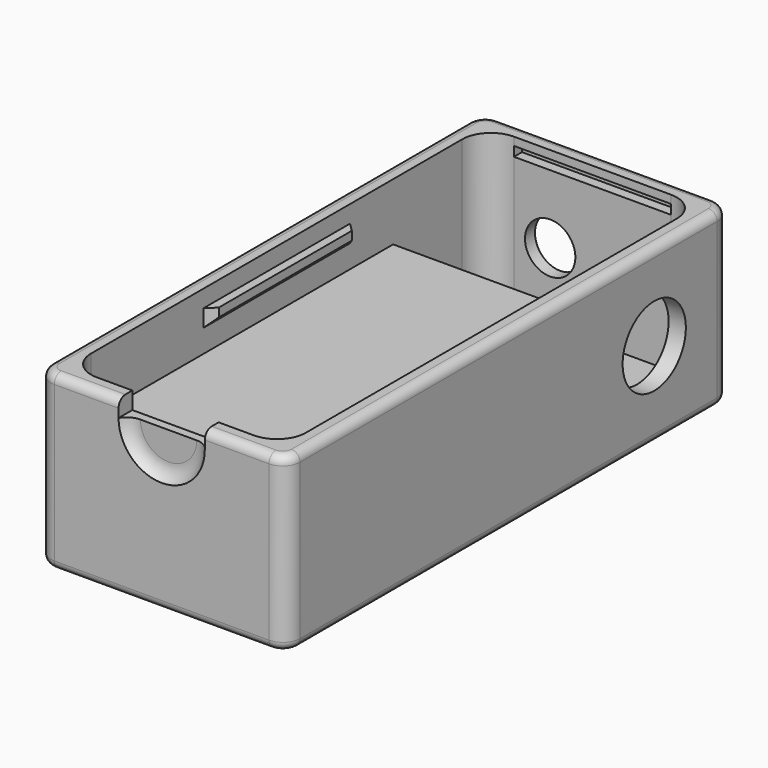
from build123d import *

# Parameters (mm, degrees)
F2_W         = 52
F2_H         = 116
F2_W_2       = 44.8
F2_H_2       = 108.8
F3_DEPTH     = 36
F4_DEPTH     = 3.6
F7_R         = 3.6
F8_R         = 5.9976
F6_R         = 5.25
F9_DEPTH     = 3.6
F5_R         = 8.25
F10_DEPTH    = 3.6
F11_W        = 18
F11_H        = 3.6
F12_DEPTH    = 3.6
F13_W        = 32.8048
F13_H        = 2
F14_DEPTH    = 2.1
F15_R        = 1.8
F6_R_2       = 12
F17_DEPTH    = 1
F18_R        = 0.5
F19_W        = 38.28
F19_H        = 3.6
F21_DEPTH    = 1.8
F20_W        = 38.28
F20_H        = 3.6
F22_DEPTH    = 1.8
F23_SIZE     = 1.79999
F25_DEPTH    = 1.8
F26_T2_ANGLE = 180
F27_W        = 41
F27_H        = 78
F28_DEPTH    = 22


# Not quite as in the source:
# - a fillet or chamfer that OpenCascade refuses, or shapes differently, is made with other operations: its cross-section is extruded or revolved along the edge and cut away or added
# - a fillet or chamfer is up to 0.001 mm smaller than in the source, because OpenCascade refuses the exact size
# - a feature of the source that left no trace in its solid (it failed there, or was rolled back) is left out


with BuildPart() as f3:
    # F2 (on Top) → F3 (new body)
    with BuildSketch(Plane.XY):
        Rectangle(F2_W, F2_H)
        Rectangle(F2_W_2, F2_H_2, mode=Mode.SUBTRACT)
    extrude(amount=F3_DEPTH)

    # F2 (on Top) → F4 (join)
    with BuildSketch(Plane.XY):
        Rectangle(F2_W_2, F2_H_2)
    extrude(amount=F4_DEPTH)

    # F7
    f7_edges = [f3.edges().sort_by_distance(p)[0] for p in [
        (26, 58, 18),
        (-26, 58, 18),
        (-26, -58, 18),
        (26, -58, 18),
    ]]
    fillet(f7_edges, radius=F7_R)

    # F8
    f8_edges = [f3.edges().sort_by_distance(p)[0] for p in [
        (-22.4, -54.4, 19.8),
        (22.4, -54.4, 19.8),
        (22.4, 54.4, 19.8),
        (-22.4, 54.4, 19.8),
    ]]
    fillet(f8_edges, radius=F8_R)

    # F6 (on face) → F9 (cut)
    with BuildSketch(Plane(origin=(0, 58, 0), x_dir=(-1, 0, 0), z_dir=(0, 1, 0))):
        with Locations((8.84, 18)):
            Circle(F6_R)
    extrude(amount=-F9_DEPTH, mode=Mode.SUBTRACT)

    # F5 (on face) → F10 (cut)
    with BuildSketch(Plane.YZ.offset(26)):
        with Locations((38, 18)):
            Circle(F5_R)
    extrude(amount=-F10_DEPTH, mode=Mode.SUBTRACT)

    # F11 (on face) → F12 (cut)
    with BuildSketch(Plane.XZ.offset(58)):
        with Locations((0, 34.2)):
            Rectangle(F11_W, F11_H)
    extrude(amount=-F12_DEPTH, mode=Mode.SUBTRACT)

    # F13 (on face) → F14 (cut)
    with BuildSketch(Plane.XZ.offset(-54.4)):
        with Locations((0, 33.3)):
            Rectangle(F13_W, F13_H)
    extrude(amount=-F14_DEPTH, mode=Mode.SUBTRACT)

    # F15
    f15_edges = [f3.edges().sort_by_distance(p)[0] for p in [
        (15.7, -58, 36),
        (24.945584, -56.945584, 36),
        (26, 0, 36),
        (-15.7, -58, 36),
        (-24.945584, -56.945584, 36),
        (-26, 0, 36),
        (-24.945584, 56.945584, 36),
        (0, 58, 36),
        (24.945584, 56.945584, 36),
        (0, -58, 0),
        (-24.945584, -56.945584, 0),
        (-26, 0, 0),
        (-24.945584, 56.945584, 0),
        (0, 58, 0),
        (24.945584, 56.945584, 0),
        (26, 0, 0),
        (24.945584, -56.945584, 0),
    ]]
    fillet(f15_edges, radius=F15_R)

    # F6 (on face) → F17 (cut)
    with BuildSketch(Plane(origin=(0, 58, 0), x_dir=(-1, 0, 0), z_dir=(0, 1, 0))):
        with Locations((8.84, 18)):
            Circle(F6_R_2)
        with Locations((8.84, 18)):
            Circle(F6_R, mode=Mode.SUBTRACT)
    extrude(amount=-F17_DEPTH, mode=Mode.SUBTRACT)

    # F18
    f18_edges = [f3.edges().sort_by_distance(p)[0] for p in [
        (0, 56.5, 34.3),
    ]]
    fillet(f18_edges, radius=F18_R)

    # F19 (on face) → F21 (join)
    with BuildSketch(Plane(origin=(22.4, 0, 0), x_dir=(0, -1, 0), z_dir=(-1, 0, 0))):
        with Locations((0, 30.6)):
            Rectangle(F19_W, F19_H)
    extrude(amount=F21_DEPTH)

    # F20 (on face) → F22 (join)
    with BuildSketch(Plane.YZ.offset(-22.4)):
        with Locations((0, 30.6)):
            Rectangle(F20_W, F20_H)
    extrude(amount=F22_DEPTH)

    # F23 (size 1.8 in the source; OpenCascade refuses exactly that, so slightly less here)
    f23_edges = [f3.edges().sort_by_distance(p)[0] for p in [
        (-20.6, -19.14, 30.6),
        (-20.6, 0, 28.8),
        (-20.6, 19.14, 30.6),
        (20.6, 19.14, 30.6),
        (20.6, 0, 28.8),
        (20.6, -19.14, 30.6),
    ]]
    chamfer(f23_edges, length=F23_SIZE)

    # F11 (on face) → F25 (cut)
    with BuildSketch(Plane.XZ.offset(58)):
        with BuildLine():
            ThreePointArc((-9, 32.4), (0, 23.4), (9, 32.4))
            Line((9, 32.4), (-9, 32.4))
        make_face()
    extrude(amount=-F25_DEPTH, mode=Mode.SUBTRACT)

    # F26: fillet of radius 3.6 on 1 edges, made by hand

    # F26_s1 → F26_t2 (revolve)
    with BuildSketch(Plane.XY.offset(32.4)):
        with BuildLine():
            ThreePointArc((-9, -58), (-7.6823085464, -56.6823085464), (-5.8823085464, -56.2))
            Line((-5.8823085464, -56.2), (-9, -56.2))
            Line((-9, -56.2), (-9, -58))
        make_face()
    revolve(axis=Axis((0, -56.2, 32.4), (0, -1, 0)), revolution_arc=F26_T2_ANGLE)


with BuildPart() as f28:
    # F27 (on face) → F28 (new body)
    with BuildSketch(Plane.XY.offset(3.6)):
        with Locations((0, -11.0006080357)):
            Rectangle(F27_W, F27_H)
    extrude(amount=F28_DEPTH)


solid = Compound([f3.part, f28.part])
